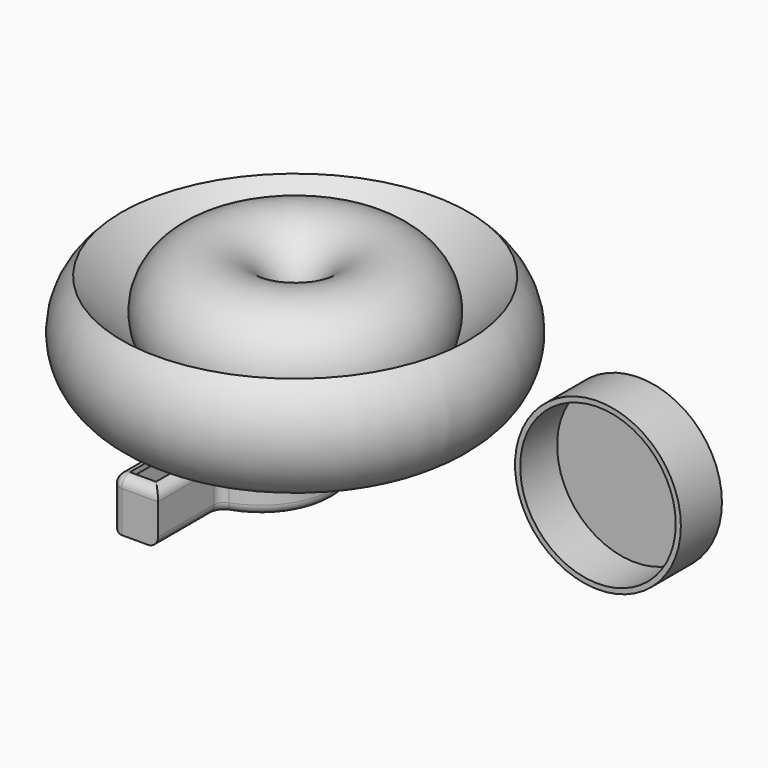
from build123d import *

# Parameters (mm, degrees)
F1_DEPTH = 25.4
F2_R     = 41.0417101423
F3_DEPTH = 25.4
F6_T     = -2.54
F7_R     = 5.08
F8_T     = -2.54


# Not quite as in the source:
# - a shell that OpenCascade refuses in one call is made with other operations: the cavity is built on its own and cut out


with BuildPart() as f1:
    # F0 (on Top) → F1 (new body)
    with BuildSketch(Plane.XY):
        with BuildLine():
            Line((-126.5921890736, -62.9820898175), (-126.5921890736, -24.4936109867))
            ThreePointArc((-126.5921890736, -24.4936109867), (-131.3958559367, 47.1175793383), (-149.6305912733, -22.2995094965))
            Line((-149.6305912733, -22.2995094965), (-149.6305912733, -62.9820898175))
            Line((-149.6305912733, -62.9820898175), (-126.5921890736, -62.9820898175))
        make_face()
    extrude(amount=F1_DEPTH)

    # F7
    f7_edges = [f1.edges().sort_by_distance(p)[0] for p in [
        (-149.630591, -42.6408, 25.4),
        (-138.11139, -62.98209, 25.4),
        (-126.592189, -43.73785, 25.4),
        (-131.395856, 47.117579, 25.4),
        (-131.395856, 47.117579, 0),
        (-126.592189, -24.493611, 12.7),
        (-149.630591, -62.98209, 12.7),
        (-149.630591, -22.299509, 12.7),
        (-149.630591, -42.6408, 0),
        (-126.592189, -43.73785, 0),
    ]]
    fillet(f7_edges, radius=F7_R)

    # F8: a shell. OpenCascade refuses it in one call, so the cavity is built on its own and cut out:
    # the body offset inwards by the wall thickness, plus a prism from it out through each open face.
    f8_core = offset(f1.part, amount=F8_T, mode=Mode.PRIVATE)
    f8_exits = [f8_core.faces().sort_by_distance(p)[0] for p in [
        (-135.30035, 3.951627, 22.86),
    ]]
    add(f8_core, mode=Mode.SUBTRACT)
    extrude(f8_exits, amount=-F8_T, mode=Mode.SUBTRACT)


with BuildPart() as f3:
    # F2 (on Front) → F3 (new body)
    with BuildSketch(Plane.XZ):
        with Locations((40.7689958811, 52.0099699497)):
            Circle(F2_R)
    extrude(amount=-F3_DEPTH)

    # F6
    f6_openings = [f3.faces().sort_by_distance(p)[0] for p in [
        (40.768996, 0, 52.00997),
    ]]
    offset(amount=F6_T, openings=f6_openings)


with BuildPart() as f5:
    # F4 (on Front) → F5 (revolve)
    with BuildSketch(Plane.XZ):
        with BuildLine():
            ThreePointArc((-45.9669940174, 74.5848789811), (-88.6373376907, 106.2971513586), (-73.108561337, 55.4514676332))
            ThreePointArc((-73.108561337, 55.4514676332), (-24.1910397784, 49.5137816107), (-23.2225875779, 98.7808307518))
            Line((-23.2225875779, 98.7808307518), (-45.9669940174, 74.5848789811))
        make_face()
    revolve(axis=Axis((-109.0912073851, 0, 83.1956714392), (0, 0, -1)))


solid = Compound([f1.part, f3.part, f5.part])
